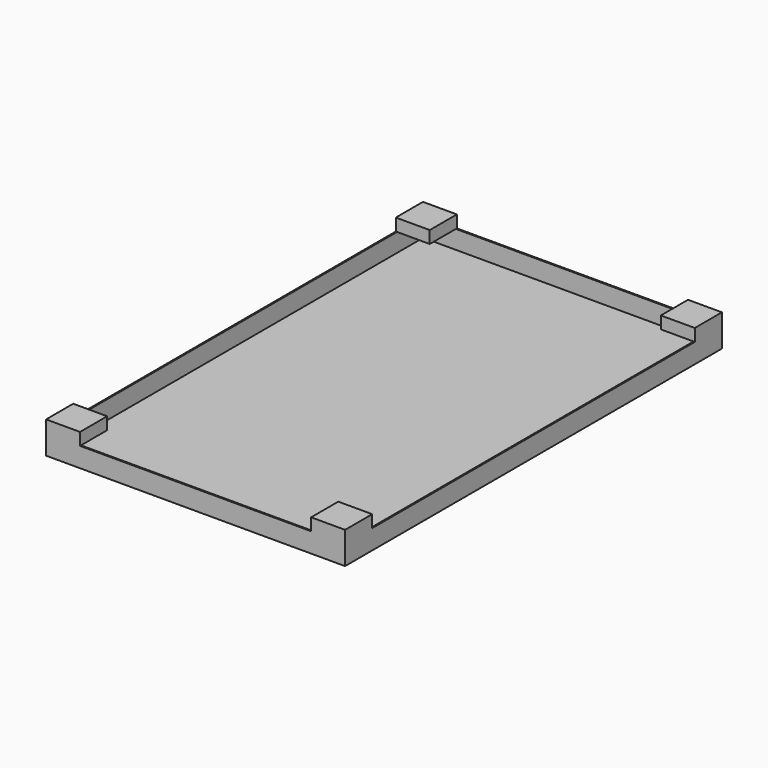
from build123d import *

# Parameters (mm, degrees)
F0_W     = 608
F0_H     = 958
F1_DEPTH = 65
F3_DEPTH = 25
F4_T     = -2.5


# Not quite as in the source:
# - a shell that OpenCascade refuses in one call is made with other operations: the cavity is built on its own and cut out


with BuildPart() as f1:
    # F0 (on Top) → F1 (new body)
    with BuildSketch(Plane.XY):
        Rectangle(F0_W, F0_H)
    extrude(amount=F1_DEPTH)

    # F2 (on face) → F3 (cut)
    with BuildSketch(Plane.XY.offset(65)):
        Polygon((235, 533.0333780003), (-235, 533.0333780003), (-235, 410), (-362.3474363838, 410), (-362.3474363838, -410), (-235, -410), (-235, -557.4594508362), (235, -557.4594508362), (235, -410), (358.7432372559, -410), (358.7432372559, 410), (235, 410), align=None)
    extrude(amount=-F3_DEPTH, mode=Mode.SUBTRACT)

    # F4: a shell. OpenCascade refuses it in one call, so the cavity is built on its own and cut out:
    # the body offset inwards by the wall thickness, plus a prism from it out through each open face.
    f4_core = offset(f1.part, amount=F4_T, kind=Kind.INTERSECTION, mode=Mode.PRIVATE)
    f4_exits = [f4_core.faces().sort_by_distance(p)[0] for p in [
        (0, 0, 37.5),
    ]]
    add(f4_core, mode=Mode.SUBTRACT)
    extrude(f4_exits, amount=-F4_T, mode=Mode.SUBTRACT)


solid = f1.part
